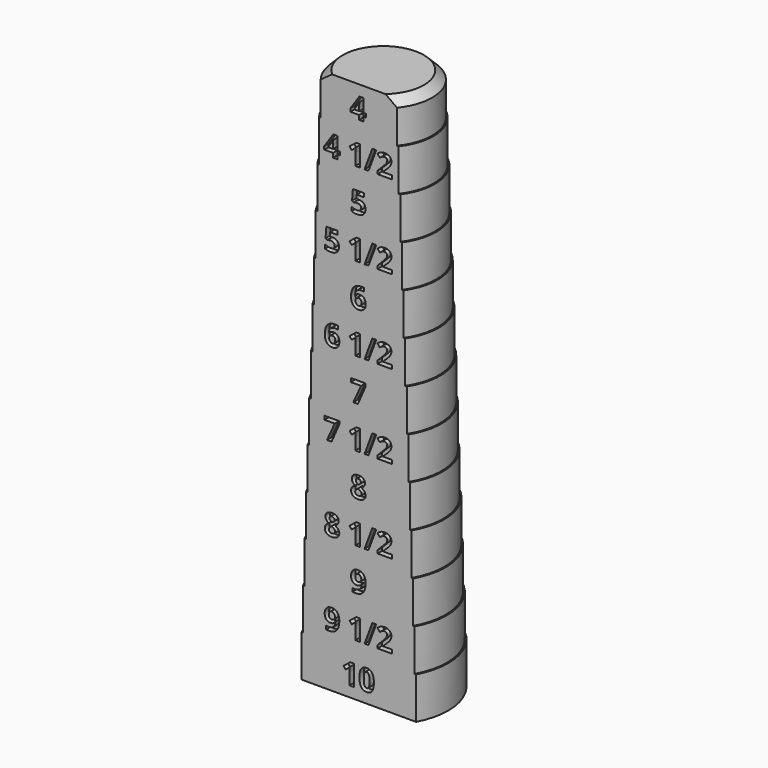
from build123d import *

# Parameters (mm, degrees)
F0_W         = 7.4422
F0_H         = 6.35
F2_SIZE      = 1.27
F6_DEPTH     = 82.551
F4_TEXT_SIZE = 4.4097222222
F7_DEPTH     = 6.35


# Not quite as in the source:
# - Text() gives the source's letters only with a copy of the font that has no kerning and outlines rounded to 1/6400 em; it was checked with that copy


with BuildPart() as f1:
    # F0 (on Front) → F1 (revolve)
    with BuildSketch(Plane.XZ):
        Polygon((0, 6.35), (0, 0), (9.8806, 0), (9.8806, 6.35), (9.6774, 6.35), align=None)
        Polygon((0, 12.7), (0, 6.35), (9.6774, 6.35), (9.6774, 12.7), (9.4742, 12.7), align=None)
        Polygon((0, 19.05), (0, 12.7), (9.4742, 12.7), (9.4742, 19.05), (9.271, 19.05), align=None)
        Polygon((0, 25.4), (0, 19.05), (9.271, 19.05), (9.271, 25.4), (9.0678, 25.4), align=None)
        Polygon((0, 31.75), (0, 25.4), (9.0678, 25.4), (9.0678, 31.75), (8.8646, 31.75), align=None)
        Polygon((0, 38.1), (0, 31.75), (8.8646, 31.75), (8.8646, 38.1), (8.6614, 38.1), align=None)
        Polygon((0, 44.45), (0, 38.1), (8.6614, 38.1), (8.6614, 44.45), (8.4582, 44.45), align=None)
        Polygon((0, 50.8), (0, 44.45), (8.4582, 44.45), (8.4582, 50.8), (8.255, 50.8), align=None)
        Polygon((0, 57.15), (0, 50.8), (8.255, 50.8), (8.255, 57.15), (8.0518, 57.15), align=None)
        Polygon((0, 63.5), (0, 57.15), (8.0518, 57.15), (8.0518, 63.5), (7.8486, 63.5), align=None)
        Polygon((0, 69.85), (0, 63.5), (7.8486, 63.5), (7.8486, 69.85), (7.6454, 69.85), align=None)
        Polygon((0, 76.2), (0, 69.85), (7.6454, 69.85), (7.6454, 76.2), (7.4422, 76.2), align=None)
        with Locations((3.7211, 79.375)):
            Rectangle(F0_W, F0_H)
    revolve(axis=Axis((0, 0, 41.275), (0, 0, 1)))

    # F2
    f2_edges = [f1.edges().sort_by_distance(p)[0] for p in [
        (-7.4422, 0, 82.55),
    ]]
    chamfer(f2_edges, length=F2_SIZE)

    # F5 (on face) → F6 (cut, through all)
    with BuildSketch(Plane.XY.offset(82.55)):
        with BuildLine():
            Line((-4.0428434253, -4.6638471114), (-12.7, -4.6638471114))
            Line((-12.7, -4.6638471114), (-12.7, -10.1248471114))
            Line((-12.7, -10.1248471114), (12.7, -10.1248471114))
            Line((12.7, -10.1248471114), (12.7, -4.6638471114))
            Line((12.7, -4.6638471114), (4.0428434253, -4.6638471114))
            ThreePointArc((4.0428434253, -4.6638471114), (0, -6.1722), (-4.0428434253, -4.6638471114))
        make_face()
        with BuildLine():
            Line((4.0428434253, -4.6638471114), (-4.0428434253, -4.6638471114))
            ThreePointArc((-4.0428434253, -4.6638471114), (0, -6.1722), (4.0428434253, -4.6638471114))
        make_face()
    extrude(amount=-F6_DEPTH, mode=Mode.SUBTRACT)

    # F4 (on offset) → F7 (cut)
    with BuildSketch(Plane.XZ.offset(10.16)):
        with Locations((-2.5814100477, 1.5875)):
            Text('10', F4_TEXT_SIZE, font='Open Sans', font_style=FontStyle.BOLD, text_align=(TextAlign.LEFT, TextAlign.BOTTOM))
        with Locations((-5.3323187934, 7.9375)):
            Text('9 1/2', F4_TEXT_SIZE, font='Open Sans', font_style=FontStyle.BOLD, text_align=(TextAlign.LEFT, TextAlign.BOTTOM))
        with Locations((-1.324983724, 14.2875)):
            Text('9', F4_TEXT_SIZE, font='Open Sans', font_style=FontStyle.BOLD, text_align=(TextAlign.LEFT, TextAlign.BOTTOM))
        with Locations((-5.3323187934, 20.6375)):
            Text('8 1/2', F4_TEXT_SIZE, font='Open Sans', font_style=FontStyle.BOLD, text_align=(TextAlign.LEFT, TextAlign.BOTTOM))
        with Locations((-1.324983724, 26.9875)):
            Text('8', F4_TEXT_SIZE, font='Open Sans', font_style=FontStyle.BOLD, text_align=(TextAlign.LEFT, TextAlign.BOTTOM))
        with Locations((-5.3323187934, 33.3375)):
            Text('7 1/2', F4_TEXT_SIZE, font='Open Sans', font_style=FontStyle.BOLD, text_align=(TextAlign.LEFT, TextAlign.BOTTOM))
        with Locations((-1.3315294054, 39.6875)):
            Text('7', F4_TEXT_SIZE, font='Open Sans', font_style=FontStyle.BOLD, text_align=(TextAlign.LEFT, TextAlign.BOTTOM))
        with Locations((-5.3323187934, 46.0375)):
            Text('6 1/2', F4_TEXT_SIZE, font='Open Sans', font_style=FontStyle.BOLD, text_align=(TextAlign.LEFT, TextAlign.BOTTOM))
        with Locations((-1.3315294054, 52.3875)):
            Text('6', F4_TEXT_SIZE, font='Open Sans', font_style=FontStyle.BOLD, text_align=(TextAlign.LEFT, TextAlign.BOTTOM))
        with Locations((-5.3323187934, 58.7375)):
            Text('5 1/2', F4_TEXT_SIZE, font='Open Sans', font_style=FontStyle.BOLD, text_align=(TextAlign.LEFT, TextAlign.BOTTOM))
        with Locations((-1.3025906033, 65.0875)):
            Text('5', F4_TEXT_SIZE, font='Open Sans', font_style=FontStyle.BOLD, text_align=(TextAlign.LEFT, TextAlign.BOTTOM))
        with Locations((-5.3323187934, 71.4375)):
            Text('4 1/2', F4_TEXT_SIZE, font='Open Sans', font_style=FontStyle.BOLD, text_align=(TextAlign.LEFT, TextAlign.BOTTOM))
        with Locations((-1.3670138889, 77.7875)):
            Text('4', F4_TEXT_SIZE, font='Open Sans', font_style=FontStyle.BOLD, text_align=(TextAlign.LEFT, TextAlign.BOTTOM))
    extrude(amount=-F7_DEPTH, mode=Mode.SUBTRACT)


solid = f1.part
